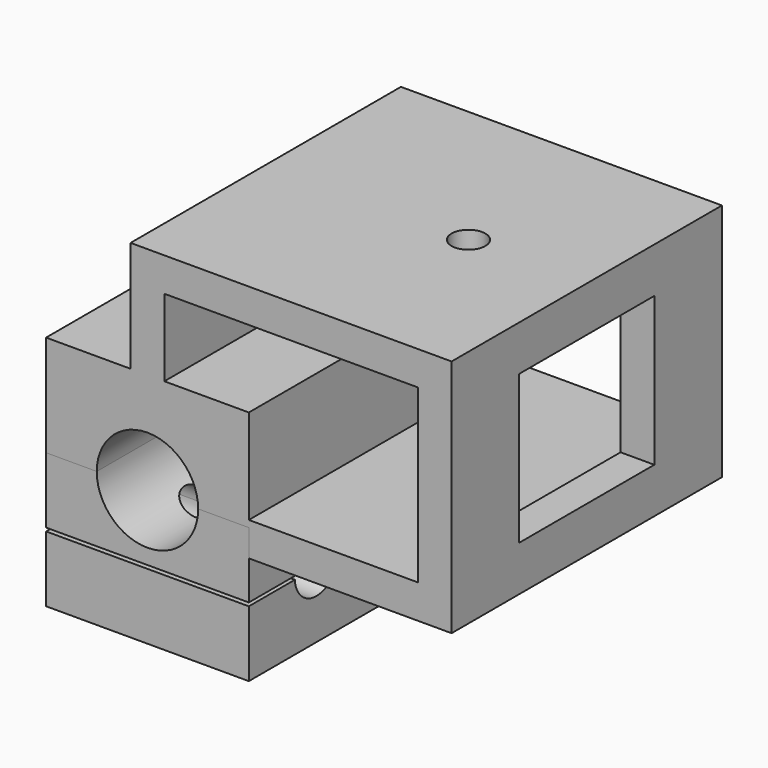
from build123d import *

# Parameters (mm, degrees)
F0_W           = 30
F0_H           = 15
F1_DEPTH       = 25
F2_R           = 7.5
F3_DEPTH       = 50.001
F4_R           = 2.5
F5_DEPTH       = 10
F6_W           = 30
F6_H           = 50
F7_DEPTH       = 20
F8_R           = 7.5
F9_DEPTH       = 50.001
F10_R          = 2.5
F11_DEPTH      = 15
F12_R          = 4
F13_DEPTH      = 30.001
F15_DEPTH      = 30.0010001
F17_DEPTH      = 25
F18_R          = 2.5
F19_DEPTH      = 21.001
F19_DEPTH_BACK = 30.401
F20_W          = 25
F20_H          = 22
F21_DEPTH      = 5


with BuildPart() as f1:
    # F0 (on Front) → F1 (new body, symmetric)
    with BuildSketch(Plane.XZ):
        with Locations((0, 7.5)):
            Rectangle(F0_W, F0_H)
    extrude(amount=F1_DEPTH, both=True)

    # F2 (on face) → F3 (cut, through all)
    with BuildSketch(Plane.XZ.offset(25)):
        Circle(F2_R)
    extrude(amount=-F3_DEPTH, mode=Mode.SUBTRACT)

    # F4 (on face) → F5 (cut)
    with BuildSketch(Plane(origin=(0, 0, 0), x_dir=(1, 0, 0), z_dir=(0, 0, -1))):
        with Locations((-11.25, 20)):
            Circle(F4_R)
        with Locations((-11.25, -20)):
            Circle(F4_R)
        with Locations((11.25, 20)):
            Circle(F4_R)
        with Locations((11.25, -20)):
            Circle(F4_R)
    extrude(amount=-F5_DEPTH, mode=Mode.SUBTRACT)

    # F16 (on Front) → F17 (join, symmetric)
    with BuildSketch(Plane.XZ):
        Polygon((15, 1), (15, -4), (45, -4), (45, 31.4), (-2.5, 31.4), (-2.5, 15), (2.5, 15), (2.5, 26.4), (40, 26.4), (40, 1), align=None)
    extrude(amount=F17_DEPTH, both=True)

    # F18 (on face) → F19 (cut, two sides)
    with BuildSketch(Plane.XY.offset(1)) as f19_sk:
        with Locations((27.5, 0)):
            Circle(F18_R)
    extrude(amount=-F19_DEPTH, mode=Mode.SUBTRACT)
    extrude(f19_sk.sketch, amount=F19_DEPTH_BACK, mode=Mode.SUBTRACT)

    # F20 (on face) → F21 (cut, through all)
    with BuildSketch(Plane.YZ.offset(45)):
        with Locations((0, 13.7)):
            Rectangle(F20_W, F20_H)
    extrude(amount=-F21_DEPTH, mode=Mode.SUBTRACT)


with BuildPart() as f7:
    # F6 (on face) → F7 (new body)
    with BuildSketch(Plane(origin=(0, 0, 0), x_dir=(1, 0, 0), z_dir=(0, 0, -1))):
        Rectangle(F6_W, F6_H)
    extrude(amount=F7_DEPTH)

    # F8 (on face) → F9 (cut, through all)
    with BuildSketch(Plane.XZ.offset(25)):
        Circle(F8_R)
    extrude(amount=-F9_DEPTH, mode=Mode.SUBTRACT)

    # F10 (on face) → F11 (cut)
    with BuildSketch(Plane(origin=(0, 0, -20), x_dir=(1, 0, 0), z_dir=(0, 0, -1))):
        with Locations((-11.25, 20)):
            Circle(F10_R)
        with Locations((11.25, 20)):
            Circle(F10_R)
        with Locations((11.25, -20)):
            Circle(F10_R)
        with Locations((-11.25, -20)):
            Circle(F10_R)
    extrude(amount=-F11_DEPTH, mode=Mode.SUBTRACT)

    # F12 (on face) → F13 (cut, through all)
    with BuildSketch(Plane.YZ.offset(15)):
        with Locations((-12.5, -10)):
            Circle(F12_R)
        with Locations((12.5, -10)):
            Circle(F12_R)
    extrude(amount=-F13_DEPTH, mode=Mode.SUBTRACT)

    # F14 (on face) → F15 (cut, through all)
    with BuildSketch(Plane(origin=(-15, 0, 0), x_dir=(0, -1, 0), z_dir=(-1, 0, 0))):
        with BuildLine():
            Line((-16.4921798557, -9.75), (-25, -9.75))
            Line((-25, -9.75), (-25, -10.25))
            Line((-25, -10.25), (-16.4921798557, -10.25))
            ThreePointArc((-16.4921798557, -10.25), (-16.5, -10), (-16.4921798557, -9.75))
        make_face()
        with BuildLine():
            Line((25, -10.25), (25, -9.75))
            Line((25, -9.75), (16.4921798557, -9.75))
            ThreePointArc((16.4921798557, -9.75), (16.5, -10), (16.4921798557, -10.25))
            Line((16.4921798557, -10.25), (25, -10.25))
        make_face()
    extrude(amount=-F15_DEPTH, mode=Mode.SUBTRACT)


solid = Compound([f1.part, f7.part])
